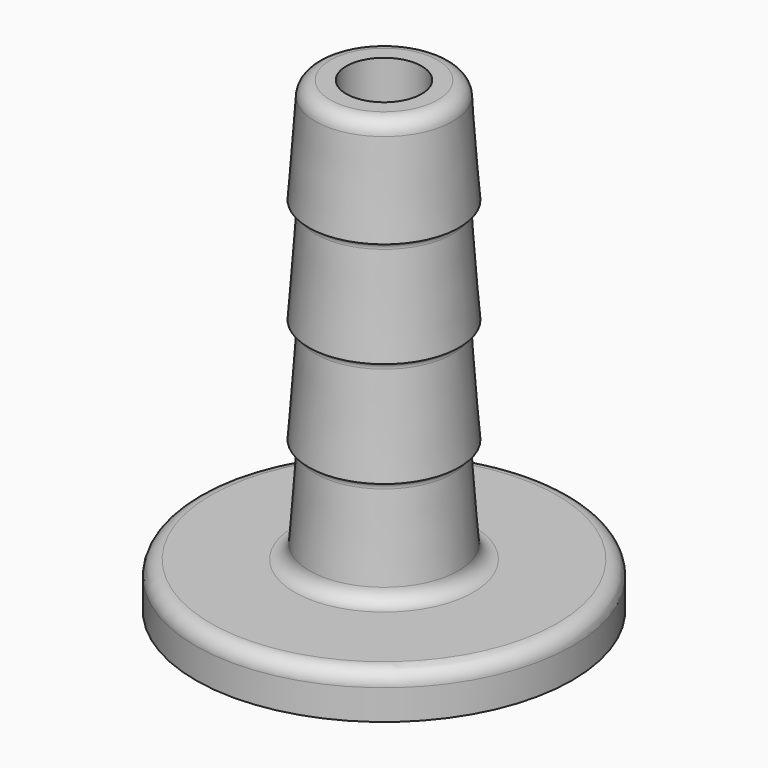
from build123d import *

# Parameters (mm, degrees)
F2_R     = 2.5
F3_DEPTH = 34
F5_R     = 1


# Not quite as in the source:
# - a fillet or chamfer that OpenCascade refuses, or shapes differently, is made with other operations: its cross-section is extruded or revolved along the edge and cut away or added


with BuildPart() as f1:
    # F0 (on Front) → F1 (revolve)
    with BuildSketch(Plane.XZ):
        Polygon((0, 28), (-4.5, 28), (-5, 21), (-4.5, 21), (-5, 14), (-4.5, 14), (-5, 7), (-4.5, 7), (-5, 0), (-12.5, 0), (-12.5, -3), (-5, -3), (-5, -6), (0, -6), align=None)
    revolve(axis=Axis((0, 0, 11), (0, 0, -1)))

    # F2 (on face) → F3 (cut, through all)
    with BuildSketch(Plane.XY.offset(28)):
        Circle(F2_R)
    extrude(amount=-F3_DEPTH, mode=Mode.SUBTRACT)

    # F4: fillet of radius 0.5 on 3 edges, made by hand

    # F4_s1 → F4_t2 (revolve)
    with BuildSketch(Plane.XZ):
        with BuildLine():
            ThreePointArc((-5, 21), (-4.6586305005, 20.8283476869), (-4.538161481, 20.4657392656))
            Line((-4.538161481, 20.4657392656), (-4.528186894, 20.4650267951))
            Line((-4.528186894, 20.4650267951), (-4.490025413, 20.9992875295))
            Line((-4.490025413, 20.9992875295), (-4.5, 21.01))
            ThreePointArc((-4.5, 21.01), (-4.75, 21.01), (-4.9992621834, 21.0099727442))
            Line((-4.9992621834, 21.0099727442), (-5, 21))
        make_face()
    revolve(axis=Axis((0, 0, 21), (0, 0, -1)))

    # F4_s3 → F4_t4 (revolve)
    with BuildSketch(Plane.XZ):
        with BuildLine():
            ThreePointArc((-5, 14), (-4.6586305005, 13.8283476869), (-4.538161481, 13.4657392656))
            Line((-4.538161481, 13.4657392656), (-4.528186894, 13.4650267951))
            Line((-4.528186894, 13.4650267951), (-4.490025413, 13.9992875295))
            Line((-4.490025413, 13.9992875295), (-4.5, 14.01))
            ThreePointArc((-4.5, 14.01), (-4.75, 14.01), (-4.9992621834, 14.0099727442))
            Line((-4.9992621834, 14.0099727442), (-5, 14))
        make_face()
    revolve(axis=Axis((0, 0, 14), (0, 0, -1)))

    # F4_s5 → F4_t6 (revolve)
    with BuildSketch(Plane.XZ):
        with BuildLine():
            ThreePointArc((-5, 7), (-4.6586305005, 6.8283476869), (-4.538161481, 6.4657392656))
            Line((-4.538161481, 6.4657392656), (-4.528186894, 6.4650267951))
            Line((-4.528186894, 6.4650267951), (-4.490025413, 6.9992875295))
            Line((-4.490025413, 6.9992875295), (-4.5, 7.01))
            ThreePointArc((-4.5, 7.01), (-4.75, 7.01), (-4.9992621834, 7.0099727442))
            Line((-4.9992621834, 7.0099727442), (-5, 7))
        make_face()
    revolve(axis=Axis((0, 0, 7), (0, 0, -1)))

    # F5
    f5_edges = [f1.edges().sort_by_distance(p)[0] for p in [
        (4.5, 0, 28),
        (5, 0, 0),
        (5, 0, -6),
        (12.5, 0, 0),
    ]]
    fillet(f5_edges, radius=F5_R)


solid = f1.part
